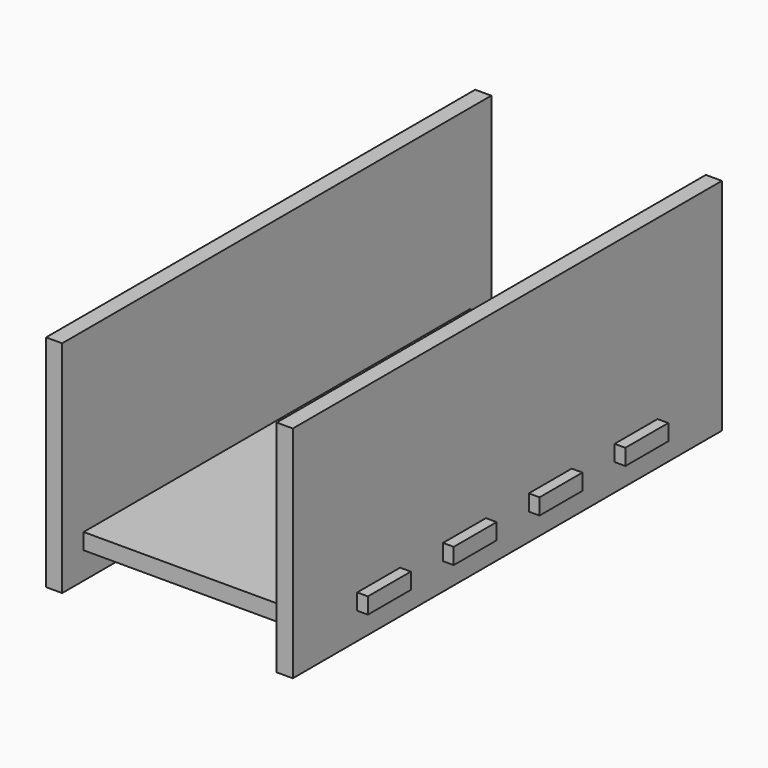
from build123d import *

# Parameters (mm, degrees)
F2_W     = 5
F2_H     = 10
F3_DEPTH = 3
F4_W     = 10
F4_H     = 3
F5_DEPTH = 23
F6_DEPTH = 20


with BuildPart() as f3:
    # F2 (on Top) → F3 (new body)
    with BuildSketch(Plane.XY):
        Polygon((-20, -45), (20, -45), (20, -35), (20, -25), (20, -15), (20, -5), (20, 5), (20, 15), (20, 25), (20, 35), (20, 45), (-20, 45), (-20, 35), (-20, 25), (-20, 15), (-20, 5), (-20, -5), (-20, -15), (-20, -25), (-20, -35), align=None)
        with Locations((-22.5, 10)):
            Rectangle(F2_W, F2_H)
        with Locations((-22.5, -10)):
            Rectangle(F2_W, F2_H)
        with Locations((-22.5, -30)):
            Rectangle(F2_W, F2_H)
        with Locations((-22.5, 30)):
            Rectangle(F2_W, F2_H)
        with Locations((22.5, 30)):
            Rectangle(F2_W, F2_H)
        with Locations((22.5, 10)):
            Rectangle(F2_W, F2_H)
        with Locations((22.5, -10)):
            Rectangle(F2_W, F2_H)
        with Locations((22.5, -30)):
            Rectangle(F2_W, F2_H)
    extrude(amount=-F3_DEPTH)


with BuildPart() as f5:
    # F4 (on Right) → F5 (new body, symmetric)
    with BuildSketch(Plane.YZ):
        Polygon((50, -8), (50, 0), (50, 33), (-50, 33), (-50, -8), align=None)
        with Locations((-30, -1.5)):
            Rectangle(F4_W, F4_H, mode=Mode.SUBTRACT)
        with Locations((-10, -1.5)):
            Rectangle(F4_W, F4_H, mode=Mode.SUBTRACT)
        with Locations((10, -1.5)):
            Rectangle(F4_W, F4_H, mode=Mode.SUBTRACT)
        with Locations((30, -1.5)):
            Rectangle(F4_W, F4_H, mode=Mode.SUBTRACT)
    extrude(amount=F5_DEPTH, both=True)

    # F4 (on Right) → F6 (cut, symmetric)
    with BuildSketch(Plane.YZ):
        Polygon((50, -8), (50, 0), (50, 33), (-50, 33), (-50, -8), align=None)
        with Locations((-30, -1.5)):
            Rectangle(F4_W, F4_H, mode=Mode.SUBTRACT)
        with Locations((-10, -1.5)):
            Rectangle(F4_W, F4_H, mode=Mode.SUBTRACT)
        with Locations((10, -1.5)):
            Rectangle(F4_W, F4_H, mode=Mode.SUBTRACT)
        with Locations((30, -1.5)):
            Rectangle(F4_W, F4_H, mode=Mode.SUBTRACT)
    extrude(amount=F6_DEPTH, both=True, mode=Mode.SUBTRACT)


solid = Compound([f3.part, f5.part])
